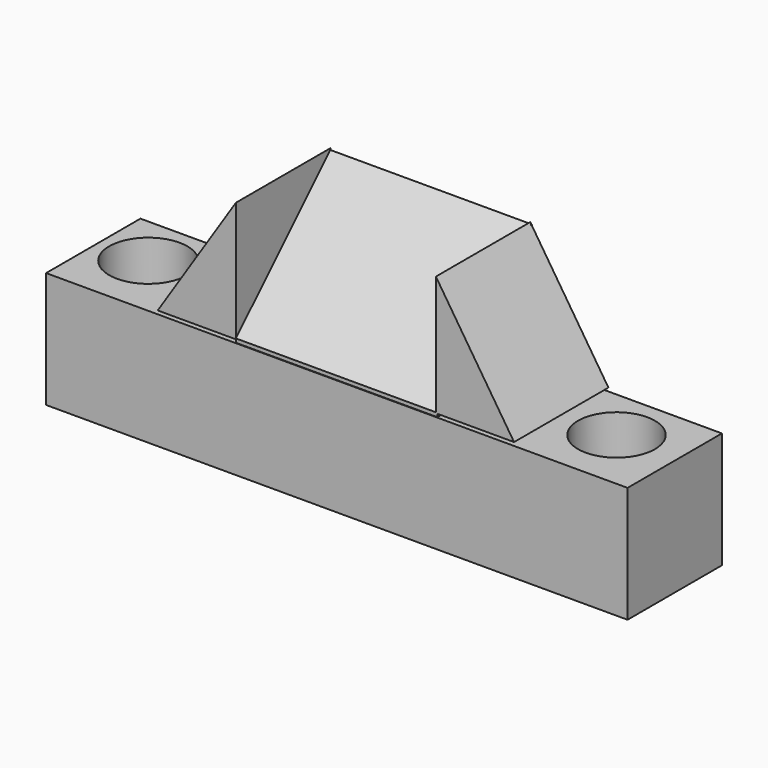
from build123d import *

# Parameters (mm, degrees)
F0_W     = 93.9071848989
F0_H     = 18.754452467
F1_DEPTH = 19.05
F2_R     = 6.2123744746
F2_R_2   = 6.3169870481
F3_DEPTH = 25.4
F4_W     = 32.5382091105
F4_H     = 19.6686182171
F5_DEPTH = 19.05
F6_SIZE  = 19.04999
F8_DEPTH = 19.05


# Not quite as in the source:
# - a fillet or chamfer is up to 0.001 mm smaller than in the source, because OpenCascade refuses the exact size


with BuildPart() as f1:
    # F0 (on Front) → F1 (new body)
    with BuildSketch(Plane.XZ):
        with Locations((2.6984810829, 9.3772262335)):
            Rectangle(F0_W, F0_H)
    extrude(amount=F1_DEPTH)

    # F2 (on Top) → F3 (cut)
    with BuildSketch(Plane.XY):
        with Locations((39.5327657461, -8.6351428181)):
            Circle(F2_R)
        with Locations((-36.2945869565, -8.3652948961)):
            Circle(F2_R_2)
    extrude(amount=F3_DEPTH, mode=Mode.SUBTRACT)


with BuildPart() as f5:
    # F4 (on Front) → F5 (new body)
    with BuildSketch(Plane.XZ):
        with Locations((2.6710461825, 28.6530507728)):
            Rectangle(F4_W, F4_H)
    extrude(amount=F5_DEPTH)

    # F6 (size 19.05 in the source; OpenCascade refuses exactly that, so slightly less here)
    f6_edges = [f5.edges().sort_by_distance(p)[0] for p in [
        (2.671046, -19.05, 38.48736),
    ]]
    chamfer(f6_edges, length=F6_SIZE)

    # F7 (on Front) → F8 (join)
    with BuildSketch(Plane.XZ):
        Polygon((31.3240997493, 19.3043854088), (18.6973288655, 38.7301817536), (18.6973288655, 19.3043854088), align=None)
        Polygon((-13.5980583727, 19.3043854088), (-13.5980583727, 38.7301817536), (-26.2248255312, 19.3043854088), align=None)
    extrude(amount=F8_DEPTH)


solid = Compound([f1.part, f5.part])
